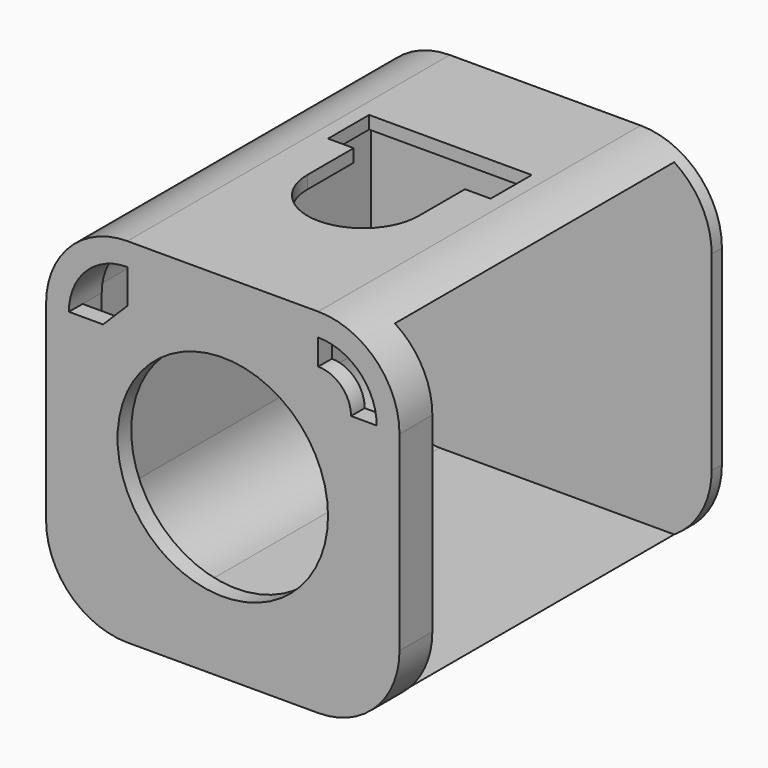
from build123d import *

# Parameters (mm, degrees)
F1_DEPTH     = 43.6
F2_DEPTH     = 4
F3_T1_DEPTH  = 22.3
F3_T6_ANGLE  = 90
F3_S7_R      = 8
F3_T8_DEPTH  = 7
F3_T12_DEPTH = 22.3
F3_T17_ANGLE = 90
F3_S18_R     = 8
F3_T19_DEPTH = 7
F3_T23_DEPTH = 22.3
F3_T28_ANGLE = 90
F3_T33_ANGLE = 90
F3_T38_DEPTH = 22.3
F5_DEPTH     = 5
F6_R         = 12.3
F7_DEPTH     = 2
F9_DEPTH     = 1.5
F10_W        = 40.8
F10_H        = 8
F10_H_2      = 22.3
F11_DEPTH    = 10


# Not quite as in the source:
# - a fillet or chamfer that OpenCascade refuses, or shapes differently, is made with other operations: its cross-section is extruded or revolved along the edge and cut away or added


with BuildPart() as f1:
    # F0 (on Front) → F1 (new body)
    with BuildSketch(Plane.XZ):
        with BuildLine():
            ThreePointArc((20.65, 11.15), (17.8675144213, 17.8675144213), (11.15, 20.65))
            Line((11.15, 20.65), (-11.15, 20.65))
            ThreePointArc((-11.15, 20.65), (-17.8675144213, 17.8675144213), (-20.65, 11.15))
            Line((-20.65, 11.15), (-20.65, -11.15))
            ThreePointArc((-20.65, -11.15), (-17.8675144213, -17.8675144213), (-11.15, -20.65))
            Line((-11.15, -20.65), (11.15, -20.65))
            ThreePointArc((11.15, -20.65), (17.8675144213, -17.8675144213), (20.65, -11.15))
            Line((20.65, -11.15), (20.65, 11.15))
        make_face()
        with BuildLine():
            Line((-11.15, 19.15), (11.15, 19.15))
            ThreePointArc((11.15, 19.15), (16.8068542495, 16.8068542495), (19.15, 11.15))
            Line((19.15, 11.15), (19.15, -11.15))
            ThreePointArc((19.15, -11.15), (16.8068542495, -16.8068542495), (11.15, -19.15))
            Line((11.15, -19.15), (-11.15, -19.15))
            ThreePointArc((-11.15, -19.15), (-16.8068542495, -16.8068542495), (-19.15, -11.15))
            Line((-19.15, -11.15), (-19.15, 11.15))
            ThreePointArc((-19.15, 11.15), (-16.8068542495, 16.8068542495), (-11.15, 19.15))
        make_face(mode=Mode.SUBTRACT)
    extrude(amount=-F1_DEPTH)

    # F0 (on Front) → F2 (join)
    with BuildSketch(Plane.XZ):
        with BuildLine():
            ThreePointArc((20.65, 11.15), (17.8675144213, 17.8675144213), (11.15, 20.65))
            Line((11.15, 20.65), (-11.15, 20.65))
            ThreePointArc((-11.15, 20.65), (-17.8675144213, 17.8675144213), (-20.65, 11.15))
            Line((-20.65, 11.15), (-20.65, -11.15))
            ThreePointArc((-20.65, -11.15), (-17.8675144213, -17.8675144213), (-11.15, -20.65))
            Line((-11.15, -20.65), (11.15, -20.65))
            ThreePointArc((11.15, -20.65), (17.8675144213, -17.8675144213), (20.65, -11.15))
            Line((20.65, -11.15), (20.65, 11.15))
        make_face()
        with BuildLine():
            Line((-11.15, 19.15), (11.15, 19.15))
            ThreePointArc((11.15, 19.15), (16.8068542495, 16.8068542495), (19.15, 11.15))
            Line((19.15, 11.15), (19.15, -11.15))
            ThreePointArc((19.15, -11.15), (16.8068542495, -16.8068542495), (11.15, -19.15))
            Line((11.15, -19.15), (-11.15, -19.15))
            ThreePointArc((-11.15, -19.15), (-16.8068542495, -16.8068542495), (-19.15, -11.15))
            Line((-19.15, -11.15), (-19.15, 11.15))
            ThreePointArc((-19.15, 11.15), (-16.8068542495, 16.8068542495), (-11.15, 19.15))
        make_face(mode=Mode.SUBTRACT)
        with BuildLine():
            ThreePointArc((19.15, 11.15), (16.8068542495, 16.8068542495), (11.15, 19.15))
            Line((11.15, 19.15), (-11.15, 19.15))
            ThreePointArc((-11.15, 19.15), (-16.8068542495, 16.8068542495), (-19.15, 11.15))
            Line((-19.15, 11.15), (-19.15, -11.15))
            ThreePointArc((-19.15, -11.15), (-16.8068542495, -16.8068542495), (-11.15, -19.15))
            Line((-11.15, -19.15), (11.15, -19.15))
            ThreePointArc((11.15, -19.15), (16.8068542495, -16.8068542495), (19.15, -11.15))
            Line((19.15, -11.15), (19.15, 11.15))
        make_face()
        with BuildLine():
            Line((-11.15, 17.985), (11.15, 17.985))
            ThreePointArc((11.15, 17.985), (15.9830748494, 15.9830748494), (17.985, 11.15))
            Line((17.985, 11.15), (17.985, -11.15))
            ThreePointArc((17.985, -11.15), (15.9830748494, -15.9830748494), (11.15, -17.985))
            Line((11.15, -17.985), (-11.15, -17.985))
            ThreePointArc((-11.15, -17.985), (-15.9830748494, -15.9830748494), (-17.985, -11.15))
            Line((-17.985, -11.15), (-17.985, 11.15))
            ThreePointArc((-17.985, 11.15), (-15.9830748494, 15.9830748494), (-11.15, 17.985))
        make_face(mode=Mode.SUBTRACT)
    extrude(amount=-F2_DEPTH)

    # F3: chamfer of 1.2 on 8 edges, made by hand

    # F3_s2 → F3_t1 (cut)
    with BuildSketch(Plane.XY.offset(-11.15)):
        Polygon((19.185, 4), (17.985, 2.8), (17.985, 4), align=None)
    extrude(amount=F3_T1_DEPTH, mode=Mode.SUBTRACT)


with BuildPart() as f3_tool4:
    # F3_s5 → F3_t6 (revolve)
    with BuildSketch(Plane.XY.offset(11.15)):
        Polygon((-19.185, 4), (-17.985, 2.8), (-17.985, 4), align=None)
    revolve(axis=Axis((-11.15, 4, 11.15), (0, 1, 0)), revolution_arc=F3_T6_ANGLE)

    # F3_s7 → F3_t8 (intersect, symmetric)
    with BuildSketch(Plane.XZ.offset(-3.4)):
        with Locations((-11.15, 11.15)):
            Circle(F3_S7_R)
    extrude(amount=F3_T8_DEPTH, both=True, mode=Mode.INTERSECT)


with BuildPart() as f1_1:
    add(f1.part)

    # F3_t3: cut F3_tool4
    add(f3_tool4.part, mode=Mode.SUBTRACT)


with BuildPart() as f3_tool10:
    # F3_s11 → F3_t12 (new body)
    with BuildSketch(Plane.XY.offset(-11.15)):
        Polygon((-19.185, 4), (-17.985, 2.8), (-17.985, 4), align=None)
    extrude(amount=F3_T12_DEPTH)

    split(bisect_by=Plane.YZ.offset(-19.15), keep=Keep.TOP)


with BuildPart() as f1_2:
    add(f1_1.part)

    # F3_t9: cut F3_tool10
    add(f3_tool10.part, mode=Mode.SUBTRACT)


with BuildPart() as f3_tool15:
    # F3_s16 → F3_t17 (revolve)
    with BuildSketch(Plane.YZ.offset(-11.15)):
        Polygon((4, -19.185), (2.8, -17.985), (4, -17.985), align=None)
    revolve(axis=Axis((-11.15, 4, -11.15), (0, 1, 0)), revolution_arc=F3_T17_ANGLE)

    # F3_s18 → F3_t19 (intersect, symmetric)
    with BuildSketch(Plane.XZ.offset(-3.4)):
        with Locations((-11.15, -11.15)):
            Circle(F3_S18_R)
    extrude(amount=F3_T19_DEPTH, both=True, mode=Mode.INTERSECT)


with BuildPart() as f1_3:
    add(f1_2.part)

    # F3_t14: cut F3_tool15
    add(f3_tool15.part, mode=Mode.SUBTRACT)


with BuildPart() as f3_tool21:
    # F3_s22 → F3_t23 (new body)
    with BuildSketch(Plane.YZ.offset(11.15)):
        Polygon((4, -19.185), (2.8, -17.985), (4, -17.985), align=None)
    extrude(amount=-F3_T23_DEPTH)

    split(bisect_by=Plane.XY.offset(-19.15), keep=Keep.TOP)


with BuildPart() as f1_4:
    add(f1_3.part)

    # F3_t20: cut F3_tool21
    add(f3_tool21.part, mode=Mode.SUBTRACT)


with BuildPart() as f3_tool26:
    # F3_s27 → F3_t28 (revolve)
    with BuildSketch(Plane.XY.offset(-11.15)):
        Polygon((19.185, 4), (17.985, 2.8), (17.985, 4), align=None)
    revolve(axis=Axis((11.15, 4, -11.15), (0, 1, 0)), revolution_arc=F3_T28_ANGLE)

    split(bisect_by=Plane.XY.offset(-19.15), keep=Keep.TOP)


with BuildPart() as f1_5:
    add(f1_4.part)

    # F3_t25: cut F3_tool26
    add(f3_tool26.part, mode=Mode.SUBTRACT)


with BuildPart() as f3_tool31:
    # F3_s32 → F3_t33 (revolve)
    with BuildSketch(Plane.YZ.offset(11.15)):
        Polygon((4, 19.185), (2.8, 17.985), (4, 17.985), align=None)
    revolve(axis=Axis((11.15, 4, 11.15), (0, 1, 0)), revolution_arc=F3_T33_ANGLE)

    split(bisect_by=Plane.XY.offset(19.15), keep=Keep.BOTTOM)


with BuildPart() as f1_6:
    add(f1_5.part)

    # F3_t30: cut F3_tool31
    add(f3_tool31.part, mode=Mode.SUBTRACT)


with BuildPart() as f3_tool36:
    # F3_s37 → F3_t38 (new body)
    with BuildSketch(Plane.YZ.offset(-11.15)):
        Polygon((4, 19.185), (2.8, 17.985), (4, 17.985), align=None)
    extrude(amount=F3_T38_DEPTH)

    split(bisect_by=Plane.XY.offset(19.15), keep=Keep.BOTTOM)


with BuildPart() as f1_7:
    add(f1_6.part)

    # F3_t35: cut F3_tool36
    add(f3_tool36.part, mode=Mode.SUBTRACT)

    # F4 (on face) → F5 (cut)
    with BuildSketch(Plane.XY.offset(20.65)):
        Polygon((-6.5, 25.25), (6.5, 25.25), (9.5, 25.25), (9.5, 31.25), (-9.5, 31.25), (-9.5, 25.25), align=None)
        with BuildLine():
            ThreePointArc((-6.5, 18.5), (0, 12), (6.5, 18.5))
            ThreePointArc((6.5, 18.5), (0, 25), (-6.5, 18.5))
        make_face()
        with BuildLine():
            ThreePointArc((-6.5, 18.5), (0, 25), (6.5, 18.5))
            Line((6.5, 18.5), (6.5, 25.25))
            Line((6.5, 25.25), (-6.5, 25.25))
            Line((-6.5, 25.25), (-6.5, 18.5))
        make_face()
    extrude(amount=-F5_DEPTH, mode=Mode.SUBTRACT)

    # F6 (on face) → F7 (join)
    with BuildSketch(Plane.XZ):
        with BuildLine():
            Line((20.65, -11.15), (20.65, 11.15))
            ThreePointArc((20.65, 11.15), (17.8675144213, 17.8675144213), (11.15, 20.65))
            Line((11.15, 20.65), (-11.15, 20.65))
            ThreePointArc((-11.15, 20.65), (-17.8675144213, 17.8675144213), (-20.65, 11.15))
            Line((-20.65, 11.15), (-20.65, -11.15))
            ThreePointArc((-20.65, -11.15), (-17.8675144213, -17.8675144213), (-11.15, -20.65))
            Line((-11.15, -20.65), (11.15, -20.65))
            ThreePointArc((11.15, -20.65), (17.8675144213, -17.8675144213), (20.65, -11.15))
        make_face()
        with BuildLine():
            ThreePointArc((11.15, 17.985), (15.9830748494, 15.9830748494), (17.985, 11.15))
            Line((17.985, 11.15), (17.985, -11.15))
            ThreePointArc((17.985, -11.15), (15.9830748494, -15.9830748494), (11.15, -17.985))
            Line((11.15, -17.985), (-11.15, -17.985))
            ThreePointArc((-11.15, -17.985), (-15.9830748494, -15.9830748494), (-17.985, -11.15))
            Line((-17.985, -11.15), (-17.985, 11.15))
            ThreePointArc((-17.985, 11.15), (-15.9830748494, 15.9830748494), (-11.15, 17.985))
            Line((-11.15, 17.985), (11.15, 17.985))
        make_face(mode=Mode.SUBTRACT)
        with BuildLine():
            Line((17.985, 11.15), (14.985, 11.15))
            ThreePointArc((14.985, 11.15), (13.8617545059, 13.8617545059), (11.15, 14.985))
            Line((11.15, 14.985), (11.15, 17.985))
            Line((11.15, 17.985), (-11.15, 17.985))
            Line((-11.15, 17.985), (-11.15, 13.985))
            Line((-11.15, 13.985), (-13.985, 11.15))
            Line((-13.985, 11.15), (-17.985, 11.15))
            Line((-17.985, 11.15), (-17.985, -11.15))
            ThreePointArc((-17.985, -11.15), (-15.9830748494, -15.9830748494), (-11.15, -17.985))
            Line((-11.15, -17.985), (11.15, -17.985))
            ThreePointArc((11.15, -17.985), (15.9830748494, -15.9830748494), (17.985, -11.15))
            Line((17.985, -11.15), (17.985, 11.15))
        make_face()
        Circle(F6_R, mode=Mode.SUBTRACT)
    extrude(amount=F7_DEPTH)

    # F8 (on face) → F9 (join)
    with BuildSketch(Plane(origin=(0, 43.6, 0), x_dir=(-1, 0, 0), z_dir=(0, 1, 0))):
        with BuildLine():
            Line((11.15, 20.65), (-11.15, 20.65))
            ThreePointArc((-11.15, 20.65), (-17.8675144213, 17.8675144213), (-20.65, 11.15))
            Line((-20.65, 11.15), (-20.65, -11.15))
            ThreePointArc((-20.65, -11.15), (-17.8675144213, -17.8675144213), (-11.15, -20.65))
            Line((-11.15, -20.65), (11.15, -20.65))
            ThreePointArc((11.15, -20.65), (17.8675144213, -17.8675144213), (20.65, -11.15))
            Line((20.65, -11.15), (20.65, 11.15))
            ThreePointArc((20.65, 11.15), (17.8675144213, 17.8675144213), (11.15, 20.65))
        make_face()
        with BuildLine():
            ThreePointArc((-19.15, 11.15), (-16.8068542495, 16.8068542495), (-11.15, 19.15))
            Line((-11.15, 19.15), (11.15, 19.15))
            ThreePointArc((11.15, 19.15), (16.8068542495, 16.8068542495), (19.15, 11.15))
            Line((19.15, 11.15), (19.15, -11.15))
            ThreePointArc((19.15, -11.15), (16.8068542495, -16.8068542495), (11.15, -19.15))
            Line((11.15, -19.15), (-11.15, -19.15))
            ThreePointArc((-11.15, -19.15), (-16.8068542495, -16.8068542495), (-19.15, -11.15))
            Line((-19.15, -11.15), (-19.15, 11.15))
        make_face(mode=Mode.SUBTRACT)
        with BuildLine():
            Line((11.15, 19.15), (-11.15, 19.15))
            ThreePointArc((-11.15, 19.15), (-16.8068542495, 16.8068542495), (-19.15, 11.15))
            Line((-19.15, 11.15), (-19.15, -11.15))
            ThreePointArc((-19.15, -11.15), (-16.8068542495, -16.8068542495), (-11.15, -19.15))
            Line((-11.15, -19.15), (11.15, -19.15))
            ThreePointArc((11.15, -19.15), (16.8068542495, -16.8068542495), (19.15, -11.15))
            Line((19.15, -11.15), (19.15, 11.15))
            ThreePointArc((19.15, 11.15), (16.8068542495, 16.8068542495), (11.15, 19.15))
        make_face()
    extrude(amount=F9_DEPTH)

    # F10 (on face) → F11 (cut)
    with BuildSketch(Plane.YZ.offset(20.65)):
        with Locations((23.2, 15.15)):
            Rectangle(F10_W, F10_H)
        with Locations((23.2, 0)):
            Rectangle(F10_W, F10_H_2)
        with Locations((23.2, -15.15)):
            Rectangle(F10_W, F10_H)
    extrude(amount=-F11_DEPTH, mode=Mode.SUBTRACT)


solid = f1_7.part
